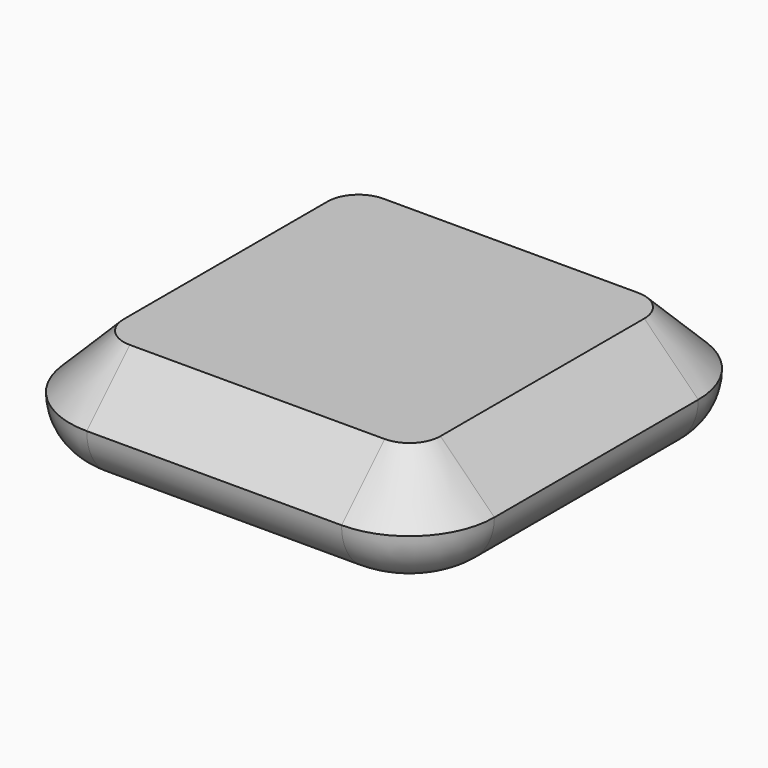
from build123d import *

# Parameters (mm, degrees)
F1_DEPTH = 25.4
F2_R     = 12.7
F3_SIZE  = 12.69999


# Not quite as in the source:
# - a fillet or chamfer is up to 0.001 mm smaller than in the source, because OpenCascade refuses the exact size


with BuildPart() as f1:
    # F0 (on Top) → F1 (new body)
    with BuildSketch(Plane.XY):
        with BuildLine():
            ThreePointArc((-50, -30), (-44.1421356237, -44.1421356237), (-30, -50))
            Line((-30, -50), (30, -50))
            ThreePointArc((30, -50), (44.1421356237, -44.1421356237), (50, -30))
            Line((50, -30), (50, 30))
            ThreePointArc((50, 30), (44.1421356237, 44.1421356237), (30, 50))
            Line((30, 50), (-30, 50))
            ThreePointArc((-30, 50), (-44.1421356237, 44.1421356237), (-50, 30))
            Line((-50, 30), (-50, -30))
        make_face()
    extrude(amount=F1_DEPTH)

    # F2
    f2_edges = [f1.edges().sort_by_distance(p)[0] for p in [
        (-44.142136, -44.142136, 0),
        (0, -50, 0),
        (44.142136, -44.142136, 0),
        (50, 0, 0),
        (44.142136, 44.142136, 0),
        (0, 50, 0),
        (-44.142136, 44.142136, 0),
        (-50, 0, 0),
    ]]
    fillet(f2_edges, radius=F2_R)

    # F3 (size 12.7 in the source; OpenCascade refuses exactly that, so slightly less here)
    f3_edges = [f1.edges().sort_by_distance(p)[0] for p in [
        (-44.142136, -44.142136, 25.4),
        (0, -50, 25.4),
        (44.142136, -44.142136, 25.4),
        (50, 0, 25.4),
        (44.142136, 44.142136, 25.4),
        (0, 50, 25.4),
        (-44.142136, 44.142136, 25.4),
        (-50, 0, 25.4),
    ]]
    chamfer(f3_edges, length=F3_SIZE)


solid = f1.part
